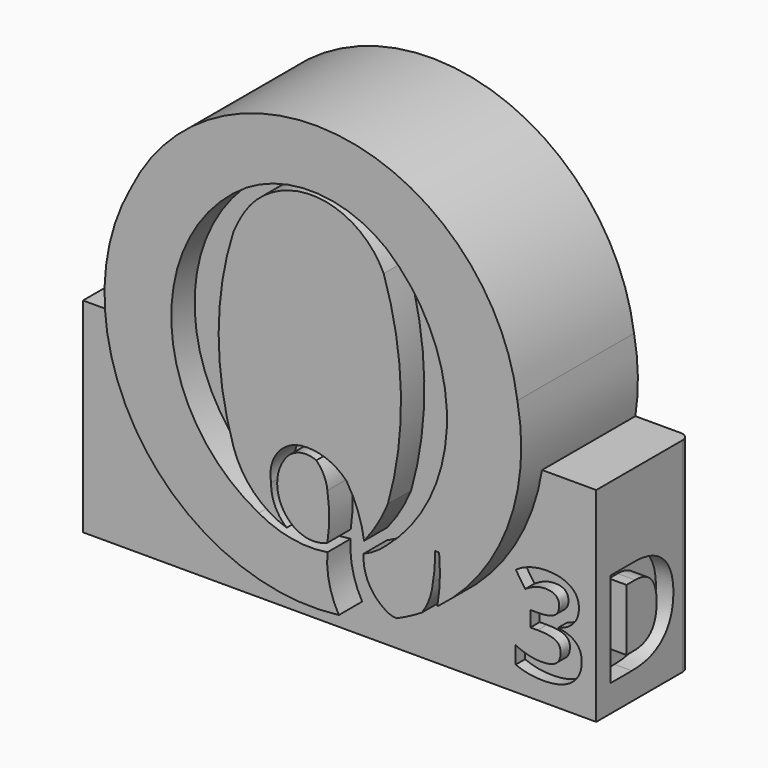
from build123d import *

# Parameters (mm, degrees)
F1_DEPTH      = 25
F5_DEPTH      = 20
F6_R          = 47.388145114
F7_DEPTH      = 35
F8_DEPTH      = 35
F9_TEXT_SIZE  = 22.7567454507
F10_DEPTH     = 3
F11_TEXT_SIZE = 22.9166666667
F12_DEPTH     = 2


# Not quite as in the source:
# - a feature of the source that left no trace in its solid (it failed there, or was rolled back) is left out
# - Text() gives the source's letters only with a copy of the font that has no kerning and outlines rounded to 1/6400 em; it was checked with that copy


with BuildPart() as f1:
    # F0 (on Front) → F1 (new body)
    with BuildSketch(Plane.XZ):
        with BuildLine():
            ThreePointArc((20.5675270408, -24.0095891058), (33.9110650067, 17.0205442488), (0, 43.6956547201))
            ThreePointArc((0, 43.6956547201), (-36.3351686492, 3.6568551313), (4.842115661, -31.3828539161))
            ThreePointArc((4.842115661, -31.3828539161), (2.4352442642, -26.4810804715), (1.9059170736, -21.0459884256))
            ThreePointArc((1.9059170736, -21.0459884256), (-4.1600004788, -20.9952833906), (-9.8727270961, -18.9550183713))
            ThreePointArc((-9.8727270961, -18.9550183713), (-24.8376639771, 4.6482965577), (-11.9922924787, 29.4688977301))
            ThreePointArc((-11.9922924787, 29.4688977301), (0.2712025373, 32.5646722625), (12.0852719992, 28.0474947466))
            ThreePointArc((12.0852719992, 28.0474947466), (22.4064776573, 5.6820438094), (12.0852719992, -16.6834071279))
            ThreePointArc((12.0852719992, -16.6834071279), (10.2163743213, -18.1512845309), (8.1104766577, -19.2524828017))
            ThreePointArc((8.1104766577, -19.2524828017), (9.1619138974, -23.770499049), (12.5694619492, -26.9179753959))
            ThreePointArc((12.5694619492, -26.9179753959), (15.3837710137, -27.0051807826), (17.7076142281, -25.4153087735))
            ThreePointArc((17.7076142281, -25.4153087735), (19.269837193, -22.7495971439), (19.9858490378, -19.7439547628))
            ThreePointArc((19.9858490378, -19.7439547628), (20.2921447856, -17.3055319325), (20.3251615167, -14.8481689394))
            Line((20.3251615167, -14.8481689394), (21.0256194399, -14.8481689394))
            Line((21.0256194399, -14.8481689394), (21.0522580892, -14.8481689394))
            ThreePointArc((21.0522580892, -14.8481689394), (21.0902538382, -15.2617533771), (21.1226022255, -15.6758177996))
            ThreePointArc((21.1226022255, -15.6758177996), (21.132303593, -19.8618351535), (20.5675270408, -24.0095891058))
        make_face()
        with BuildLine():
            ThreePointArc((21.0256194399, -14.8481689394), (21.0746144936, -15.2619343512), (21.1226022255, -15.6758177996))
            ThreePointArc((21.1226022255, -15.6758177996), (21.0902538382, -15.2617533771), (21.0522580892, -14.8481689394))
            Line((21.0522580892, -14.8481689394), (21.0256194399, -14.8481689394))
        make_face()
    extrude(amount=F1_DEPTH)



with BuildPart() as f1b:
    # F0 (on Front) → F1, piece 2 (new body)
    with BuildSketch(Plane.XZ):
        with BuildLine():
            ThreePointArc((12.268330361, -10.3936661035), (14.5129050486, 6.9410317552), (11.5593973569, 24.1691093523))
            ThreePointArc((11.5593973569, 24.1691093523), (0.054070856, 31.9757142755), (-12.3297718844, 25.6546338853))
            ThreePointArc((-12.3297718844, 25.6546338853), (-13.3290953166, 23.9329823971), (-14.1917197034, 22.1389338089))
            ThreePointArc((-14.1917197034, 22.1389338089), (-16.7424053891, 5.8726338527), (-14.1917197034, -10.3936661035))
            ThreePointArc((-14.1917197034, -10.3936661035), (-10.7371054629, -16.0907978602), (-5.083876662, -19.6167975664))
            ThreePointArc((-5.083876662, -19.6167975664), (-7.0866938375, -16.9582762129), (-7.747025229, -13.6959189549))
            ThreePointArc((-7.747025229, -13.6959189549), (-6.7687697312, -8.9761092435), (-2.6743013877, -6.4327027649))
            ThreePointArc((-2.6743013877, -6.4327027649), (1.5733205373, -6.8874333521), (5.1653617993, -9.1996425763))
            ThreePointArc((5.1653617993, -9.1996425763), (7.1251059685, -13.0735291849), (8.192373784, -17.2816800941))
            ThreePointArc((8.192373784, -17.2816800941), (10.4826039511, -13.9869422067), (12.268330361, -10.3936661035))
        make_face()
    extrude(amount=F1_DEPTH)


with BuildPart() as f1c:
    # F0 (on Front) → F1, piece 3 (new body)
    with BuildSketch(Plane.XZ):
        with BuildLine():
            ThreePointArc((-4.3943715282, -18.6494458467), (-1.3895715664, -20.0797383967), (1.9059170736, -19.6167975664))
            ThreePointArc((1.9059170736, -19.6167975664), (2.2170849753, -15.6672932208), (1.9059170736, -11.7177888751))
            ThreePointArc((1.9059170736, -11.7177888751), (1.2976371918, -9.5873136493), (0, -7.7914665453))
            ThreePointArc((0, -7.7914665453), (-3.1194388672, -7.6353877754), (-5.5577261373, -9.5873136493))
            ThreePointArc((-5.5577261373, -9.5873136493), (-6.6520631202, -14.3335387088), (-4.3943715282, -18.6494458467))
        make_face()
    extrude(amount=F1_DEPTH)


with BuildPart() as f1_1:
    add(f1.part)

    add(f1b.part)  # F5 merges F1b

    add(f1c.part)  # F5 merges F1c
    # F4 (on face) → F5 (join)
    with BuildSketch(Plane(origin=(0, 0, 0), x_dir=(-1, 0, 0), z_dir=(0, 1, 0))):
        with BuildLine():
            ThreePointArc((35.7798538129, 11.3915813367), (1.8595130932, 42.8043288316), (-34.3636036969, 14.0774071426))
            ThreePointArc((-34.3636036969, 14.0774071426), (-0.9549955614, -30.6998305937), (35.7798538129, 11.3915813367))
        make_face()
    extrude(amount=-F5_DEPTH)

    # F6 (on face) → F7 (cut)
    with BuildSketch(Plane(origin=(0, 0, 0), x_dir=(-1, 0, 0), z_dir=(0, 1, 0))):
        with Locations((0.5864036649, 5.5613326442)):
            Circle(F6_R)
        with BuildLine():
            ThreePointArc((31.8091168289, 22.930546738), (6.1793249327, -29.7270032085), (-34.4769854351, 12.424725419))
            ThreePointArc((-34.4769854351, 12.424725419), (-5.2350774941, 42.2917589206), (31.8091168289, 22.930546738))
        make_face(mode=Mode.SUBTRACT)
    extrude(amount=-F7_DEPTH, mode=Mode.SUBTRACT)

    # F3 (on Top) → F8 (join)
    with BuildSketch(Plane.XY):
        with BuildLine():
            ThreePointArc((44, -1.5), (43.5606601718, -0.4393398282), (42.5, 0))
            Line((42.5, 0), (-42.5, 0))
            ThreePointArc((-42.5, 0), (-43.5606601718, -0.4393398282), (-44, -1.5))
            Line((-44, -1.5), (-44, -20))
            Line((-44, -20), (44, -20))
            Line((44, -20), (44, -1.5))
        make_face()
    extrude(amount=-F8_DEPTH)

    # F9 (on face) → F10 (cut)
    with BuildSketch(Plane.YZ.offset(44)):
        with Locations((-19, -30.3848567245)):
            Text('D', F9_TEXT_SIZE, font='Open Sans', font_style=FontStyle.BOLD, text_align=(TextAlign.LEFT, TextAlign.BOTTOM))
    extrude(amount=-F10_DEPTH, mode=Mode.SUBTRACT)

    # F11 (on face) → F12 (cut)
    with BuildSketch(Plane.XZ.offset(20)):
        with Locations((29.3180338542, -31.5)):
            Text('3', F11_TEXT_SIZE, font='Open Sans', font_style=FontStyle.BOLD, text_align=(TextAlign.LEFT, TextAlign.BOTTOM))
    extrude(amount=-F12_DEPTH, mode=Mode.SUBTRACT)


solid = f1_1.part
